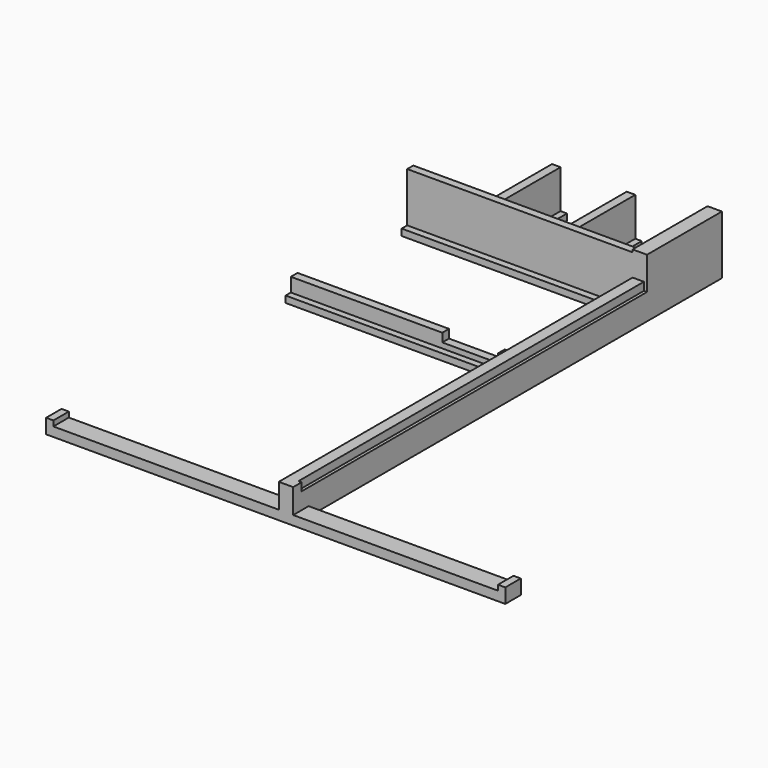
from build123d import *

# Parameters (mm, degrees)
F0_W           = 5990
F0_H           = 590
F0_W_2         = 590
F0_H_2         = 2170
F1_DEPTH       = 180
F2_W           = 395
F2_H           = 14705
F3_DEPTH       = 750
F4_W           = 395
F4_H           = 2570
F5_DEPTH       = 680
F6_W           = 85
F6_H           = 11845
F7_DEPTH       = 220
F8_W           = 6185
F8_H           = 230
F9_DEPTH       = 380
F10_W          = 1530
F10_H          = 230
F11_DEPTH      = 235
F12_W          = 6185
F12_H          = 210
F13_DEPTH      = 1060
F14_W          = 235
F14_H          = 2360
F15_DEPTH      = 1060
F16_W          = 12199.99962
F16_H          = 530
F17_DEPTH      = 255
F18_W          = 85
F18_H          = 900
F19_DEPTH      = 2570.001
F20_W          = 6185
F20_H          = 210
F21_DEPTH      = 300
F22_W          = 85
F22_H          = 2570
F23_DEPTH      = 900
F24_W          = 200.1
F24_H          = 530
F25_DEPTH      = 145.1
F25_DEPTH_BACK = 255
F26_W          = 200.5
F26_H          = 530
F27_DEPTH      = 145.5
F27_DEPTH_BACK = 255


# Not quite as in the source:
# - a feature names something its author has since deleted; it is built from what else it names


with BuildPart() as f1:
    # F0 (on Top) → F1 (new body)
    with BuildSketch(Plane.XY):
        Polygon((0, 7965), (0, 0), (590, 0), (590, 14705), (0, 14705), (0, 12535), (0, 11945), (0, 8555), align=None)
        with Locations((-2995, 8260)):
            Rectangle(F0_W, F0_H)
        Polygon((-5990, 11945), (0, 11945), (0, 12535), (-1610, 12535), (-2200, 12535), (-3660, 12535), (-4250, 12535), (-5990, 12535), align=None)
        with Locations((-3955, 13620)):
            Rectangle(F0_W_2, F0_H_2)
        with Locations((-1905, 13620)):
            Rectangle(F0_W_2, F0_H_2)
    extrude(amount=F1_DEPTH)

    # F2 (on face) → F3 (join)
    with BuildSketch(Plane.XY.offset(180)):
        with Locations((392.5, 7352.5)):
            Rectangle(F2_W, F2_H)
    extrude(amount=F3_DEPTH)

    # F4 (on face) → F5 (join)
    with BuildSketch(Plane.XY.offset(930)):
        with Locations((392.5, 13420)):
            Rectangle(F4_W, F4_H)
    extrude(amount=F5_DEPTH)

    # F6 (on face) → F7 (cut)
    with BuildSketch(Plane.XY.offset(930)):
        with Locations((547.5, 6212.5)):
            Rectangle(F6_W, F6_H)
    extrude(amount=-F7_DEPTH, mode=Mode.SUBTRACT)

    # F8 (on face) → F9 (join)
    with BuildSketch(Plane.XY.offset(180)):
        with Locations((-2897.5, 8260)):
            Rectangle(F8_W, F8_H)
    extrude(amount=F9_DEPTH)

    # F10 (on face) → F11 (cut)
    with BuildSketch(Plane.XY.offset(560)):
        with Locations((-1070, 8260)):
            Rectangle(F10_W, F10_H)
    extrude(amount=-F11_DEPTH, mode=Mode.SUBTRACT)

    # F12 (on face) → F13 (join)
    with BuildSketch(Plane.XY.offset(180)):
        with Locations((-2897.5, 12240)):
            Rectangle(F12_W, F12_H)
    extrude(amount=F13_DEPTH)

    # F14 (on face) → F15 (join, through all)
    with BuildSketch(Plane.XY.offset(180)):
        with Locations((-3955, 13525)):
            Rectangle(F14_W, F14_H)
        with Locations((-1905, 13525)):
            Rectangle(F14_W, F14_H)
    extrude(amount=F15_DEPTH)

    # F16 (on face) → F17 (join)
    with BuildSketch(Plane(origin=(0, 0, 0), x_dir=(1, 0, 0), z_dir=(0, 0, -1))):
        with Locations((109.99981, -265)):
            Rectangle(F16_W, F16_H)
    extrude(amount=-F17_DEPTH)

    # F18 (on face) → F19 (cut, through all)
    with BuildSketch(Plane.XZ.offset(-12135)):
        with Locations((547.5, 1160)):
            Rectangle(F18_W, F18_H)
    extrude(amount=-F19_DEPTH, mode=Mode.SUBTRACT)

    # F20 (on face) → F21 (join)
    with BuildSketch(Plane.XY.offset(1240)):
        with Locations((-2897.5, 12240)):
            Rectangle(F20_W, F20_H)
    extrude(amount=F21_DEPTH)

    # F22 (on face) → F23 (join, through all)
    with BuildSketch(Plane.XY.offset(710)):
        with Locations((547.5, 13420)):
            Rectangle(F22_W, F22_H)
    extrude(amount=F23_DEPTH)

    # F24 (on face) → F25 (join, two sides)
    with BuildSketch(Plane.XY.offset(255)) as f25_sk:
        with Locations((-6090.05, 265)):
            Rectangle(F24_W, F24_H)
    extrude(amount=F25_DEPTH)
    extrude(f25_sk.sketch, amount=-F25_DEPTH_BACK)

    # F26 (on face) → F27 (join, two sides)
    with BuildSketch(Plane.XY.offset(255)) as f27_sk:
        with Locations((6310.24962, 265)):
            Rectangle(F26_W, F26_H)
    extrude(amount=F27_DEPTH)
    extrude(f27_sk.sketch, amount=-F27_DEPTH_BACK)


solid = f1.part
